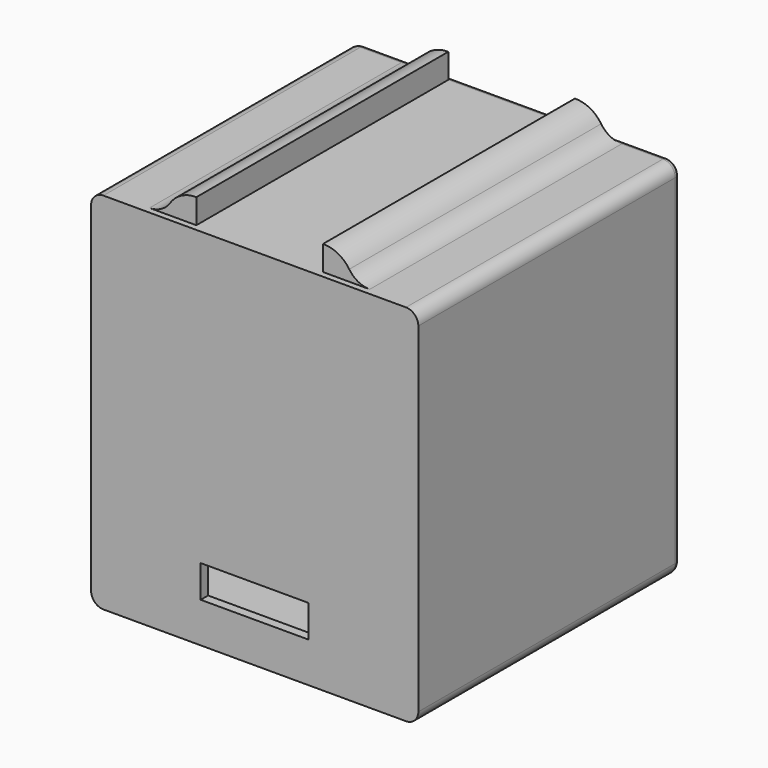
from build123d import *

# Parameters (mm, degrees)
F0_W         = 134.62
F0_H         = 134.62
F0_W_2       = 127
F0_H_2       = 127
F1_DEPTH     = 140.97
F2_W         = 134.62
F2_H         = 134.62
F3_DEPTH     = 5.08
F4_W         = 22.225
F4_H         = 13.2926666667
F5_DEPTH     = 3.81
F6_W         = 134.62
F6_H         = 134.62
F7_DEPTH     = 3.81
F8_W         = 127
F8_H         = 142.24
F9_DEPTH     = 3.81
F10_W        = 127
F10_H        = 1.27
F11_DEPTH    = 127
F12_R        = 5.08
F13_R        = 2.54
F14_W        = 12.7
F14_H        = 129.54
F15_DEPTH    = 10.16
F16_T1_DEPTH = 191.7570394667
F17_T1_DEPTH = 129.54


# Not quite as in the source:
# - a fillet or chamfer that OpenCascade refuses, or shapes differently, is made with other operations: its cross-section is extruded or revolved along the edge and cut away or added


with BuildPart() as f1:
    # F0 (on Top) → F1 (new body)
    with BuildSketch(Plane.XY):
        Rectangle(F0_W, F0_H)
        Rectangle(F0_W_2, F0_H_2, mode=Mode.SUBTRACT)
    extrude(amount=F1_DEPTH)

    # F2 (on face) → F3 (join)
    with BuildSketch(Plane.XY.offset(140.97)):
        Rectangle(F2_W, F2_H)
    extrude(amount=F3_DEPTH)

    # F4 (on face) → F5 (cut, through all)
    with BuildSketch(Plane.XZ.offset(67.31)):
        with Locations((11.1125, 19.3463333333)):
            Rectangle(F4_W, F4_H)
        with Locations((-11.1125, 19.3463333333)):
            Rectangle(F4_W, F4_H)
    extrude(amount=-F5_DEPTH, mode=Mode.SUBTRACT)

    # F6 (on face) → F7 (join)
    with BuildSketch(Plane(origin=(0, 0, 0), x_dir=(1, 0, 0), z_dir=(0, 0, -1))):
        Rectangle(F6_W, F6_H)
    extrude(amount=F7_DEPTH)

    # F8 (on face) → F9 (cut)
    with BuildSketch(Plane(origin=(0, 67.31, 0), x_dir=(-1, 0, 0), z_dir=(0, 1, 0))):
        with Locations((0, 71.12)):
            Rectangle(F8_W, F8_H)
    extrude(amount=-F9_DEPTH, mode=Mode.SUBTRACT)

    # F10 (on face) → F11 (cut, through all)
    with BuildSketch(Plane(origin=(0, 63.5, 0), x_dir=(-1, 0, 0), z_dir=(0, 1, 0))):
        with Locations((0, 141.605)):
            Rectangle(F10_W, F10_H)
    extrude(amount=-F11_DEPTH, mode=Mode.SUBTRACT)

    # F12
    f12_edges = [f1.edges().sort_by_distance(p)[0] for p in [
        (-67.31, 0, -3.81),
        (67.31, 0, -3.81),
        (67.31, 0, 146.05),
        (-67.31, 0, 146.05),
    ]]
    fillet(f12_edges, radius=F12_R)

    # F13
    f13_edges = [f1.edges().sort_by_distance(p)[0] for p in [
        (67.31, 67.31, 71.12),
        (0, 67.31, -3.81),
        (0, 67.31, 146.05),
        (-67.31, 67.31, 71.12),
        (65.822102, 67.31, 144.562102),
        (65.822102, 67.31, -2.322102),
        (-65.822102, 67.31, 144.562102),
        (-65.822102, 67.31, -2.322102),
    ]]
    fillet(f13_edges, radius=F13_R)

    # F14 (on face) → F15 (join)
    with BuildSketch(Plane.XY.offset(146.05)):
        with Locations((-32.385, 0)):
            Rectangle(F14_W, F14_H)
        with Locations((32.385, 0)):
            Rectangle(F14_W, F14_H)
    extrude(amount=F15_DEPTH)

    # F16: fillet of radius 12.7 on 2 edges, made by hand

    # F16_s2 → F16_t1 (cut)
    with BuildSketch(Plane.XZ.offset(-95.8785197333)):
        with BuildLine():
            ThreePointArc((-38.735, 146.05), (-34.3237773635, 153.3473776994), (-26.2915921067, 156.21))
            Line((-26.2915921067, 156.21), (-38.735, 156.21))
            Line((-38.735, 156.21), (-38.735, 146.05))
        make_face()
        with BuildLine():
            ThreePointArc((38.735, 146.05), (34.3237773635, 153.3473776994), (26.2915921067, 156.21))
            Line((26.2915921067, 156.21), (38.735, 156.21))
            Line((38.735, 156.21), (38.735, 146.05))
        make_face()
    extrude(amount=F16_T1_DEPTH, mode=Mode.SUBTRACT)

    # F17: fillet of radius 10.16 on 2 edges, made by hand

    # F17_s2 → F17_t1 (join)
    with BuildSketch(Plane.XZ.offset(-64.77)):
        with BuildLine():
            ThreePointArc((-36.8513807316, 150.5655555556), (-40.5097417003, 147.2497222265), (-45.2992116315, 146.05))
            Line((-45.2992116315, 146.05), (-38.735, 146.05))
            ThreePointArc((-38.735, 146.05), (-38.0126979849, 148.3993432066), (-36.8513807316, 150.5655555556))
        make_face()
        with BuildLine():
            ThreePointArc((36.8513807316, 150.5655555556), (40.5097417003, 147.2497222265), (45.2992116315, 146.05))
            Line((45.2992116315, 146.05), (38.735, 146.05))
            ThreePointArc((38.735, 146.05), (38.0126979849, 148.3993432066), (36.8513807316, 150.5655555556))
        make_face()
    extrude(amount=F17_T1_DEPTH)


solid = f1.part
